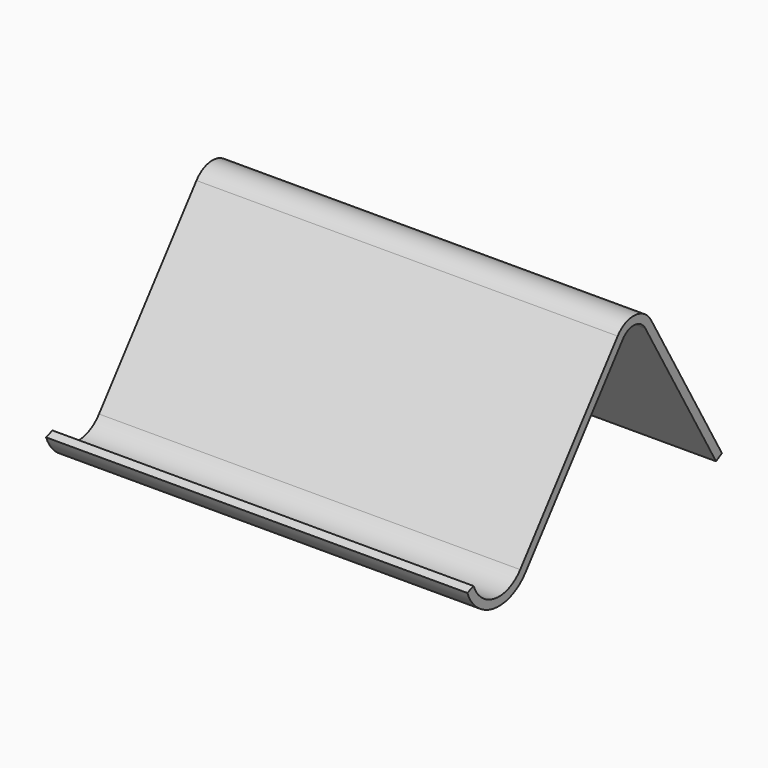
from build123d import *

# Parameters (mm, degrees)
F1_DEPTH     = 100
F2_TEXT_SIZE = 30.0344144332
F3_DEPTH     = 1


# Not quite as in the source:
# - Text() gives the source's letters only with a copy of the font that has no kerning and outlines rounded to 1/6400 em; it was checked with that copy


with BuildPart() as f1:
    # F0 (on Right) → F1 (new body)
    with BuildSketch(Plane.YZ):
        with BuildLine():
            ThreePointArc((4.4516113795, 36.3623516559), (-0.3275242067, 39.345298856), (-5.4729582171, 37.0512587965))
            Line((-5.4729582171, 37.0512587965), (-34.3901541668, 0))
            ThreePointArc((-34.3901541668, 0), (-41.9503995657, -2.9790864321), (-48.2171882592, 2.1938842745))
            Line((-48.2171882592, 2.1938842745), (-50.0972974717, 1.5118363666))
            ThreePointArc((-50.0972974717, 1.5118363666), (-42.2638116049, -4.9543770167), (-32.8135048564, -1.2305189766))
            Line((-32.8135048564, -1.2305189766), (-3.8963089066, 35.8207398199))
            ThreePointArc((-3.8963089066, 35.8207398199), (-0.4660195663, 37.3500998596), (2.7200708245, 35.3614683928))
            Line((2.7200708245, 35.3614683928), (23.7386193484, -1.000883263))
            Line((23.7386193484, -1.000883263), (25.4701599035, 0))
            Line((25.4701599035, 0), (4.4516113795, 36.3623516559))
        make_face()
    extrude(amount=F1_DEPTH)

    # F2 (on face) → F3 (join)
    with BuildSketch(Plane(origin=(0, 19.0913665344, 11.0353922565), x_dir=(-1, 0, 0), z_dir=(0, 0.8657702775, 0.5004416315))):
        with Locations((-95.5, -5.1595011607)):
            Text('Hanna', F2_TEXT_SIZE, font='Open Sans', text_align=(TextAlign.LEFT, TextAlign.BOTTOM))
    extrude(amount=F3_DEPTH)


solid = f1.part
